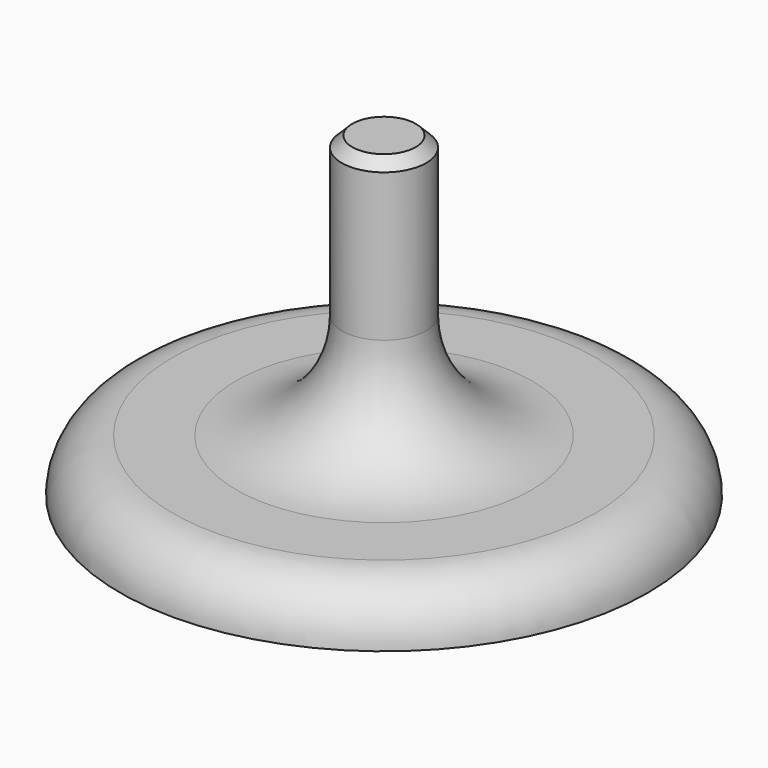
from build123d import *

# Parameters (mm, degrees)
F0_R     = 25
F2_DEPTH = 5
F1_R     = 4
F3_DEPTH = 30
F4_R     = 10
F5_R     = 4.99999
F6_SIZE  = 1


# Not quite as in the source:
# - a fillet or chamfer is up to 0.001 mm smaller than in the source, because OpenCascade refuses the exact size


with BuildPart() as f2:
    # F0 (on Top) → F2 (new body)
    with BuildSketch(Plane.XY):
        Circle(F0_R)
    extrude(amount=F2_DEPTH)

    # F1 (on face) → F3 (join)
    with BuildSketch(Plane.XY):
        Circle(F1_R)
    extrude(amount=F3_DEPTH)

    # F4
    f4_edges = [f2.edges().sort_by_distance(p)[0] for p in [
        (-4, 0, 5),
    ]]
    fillet(f4_edges, radius=F4_R)

    # F5 (radius 5 in the source; OpenCascade refuses exactly that, so slightly less here)
    f5_edges = [f2.edges().sort_by_distance(p)[0] for p in [
        (-25, 0, 5),
    ]]
    fillet(f5_edges, radius=F5_R)

    # F6
    f6_edges = [f2.edges().sort_by_distance(p)[0] for p in [
        (-4, 0, 30),
    ]]
    chamfer(f6_edges, length=F6_SIZE)


solid = f2.part
